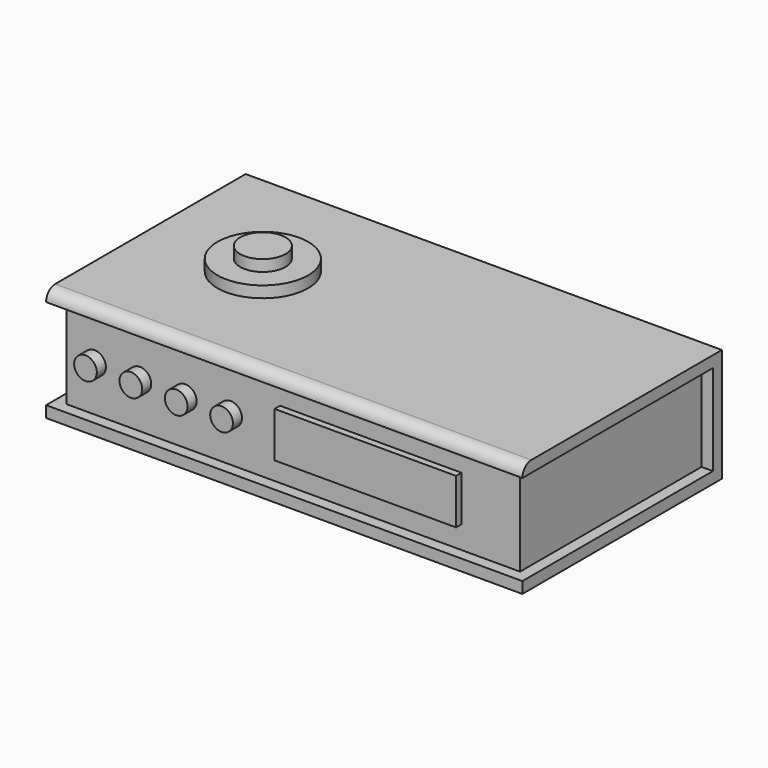
from build123d import *

# Parameters (mm, degrees)
F0_W      = 200
F0_H      = 100
F1_DEPTH  = 40
F2_W      = 210
F2_H      = 105
F2_W_2    = 200
F2_H_2    = 100
F3_DEPTH  = 5
F4_W      = 210
F4_H      = 105
F5_DEPTH  = 5
F6_W      = 210
F6_H      = 50
F7_DEPTH  = 5
F8_R      = 20
F9_DEPTH  = 5
F10_R     = 10
F11_DEPTH = 5
F12_R     = 5
F13_DEPTH = 5
F14_DEPTH = 5
F15_DEPTH = 5
F16_DEPTH = 5
F12_W     = 80
F12_H     = 20
F17_DEPTH = 3
F18_R     = 4.99999


# Not quite as in the source:
# - a fillet or chamfer is up to 0.001 mm smaller than in the source, because OpenCascade refuses the exact size


with BuildPart() as f1:
    # F0 (on Top) → F1 (new body)
    with BuildSketch(Plane.XY):
        with Locations((8.9475423098, -1.9630908966)):
            Rectangle(F0_W, F0_H)
    extrude(amount=F1_DEPTH)

    # F2 (on face) → F3 (join)
    with BuildSketch(Plane.XY.offset(40)):
        Polygon((113.9475423098, -56.9630908966), (113.9475423098, 48.0369091034), (108.9475423098, 48.0369091034), (108.9475423098, -51.9630908966), (-91.0524576902, -51.9630908966), (-91.0524576902, 48.0369091034), (-96.0524576902, 48.0369091034), (-96.0524576902, -56.9630908966), align=None)
        with Locations((8.9475423098, -4.4630908966)):
            Rectangle(F2_W, F2_H)
        with Locations((8.9475423098, -1.9630908966)):
            Rectangle(F2_W_2, F2_H_2)
    extrude(amount=F3_DEPTH)

    # F4 (on face) → F5 (join)
    with BuildSketch(Plane(origin=(0, 0, 0), x_dir=(1, 0, 0), z_dir=(0, 0, -1))):
        with Locations((8.9475423098, 4.4630908966)):
            Rectangle(F4_W, F4_H)
    extrude(amount=F5_DEPTH)

    # F6 (on face) → F7 (join)
    with BuildSketch(Plane(origin=(0, 48.0369091034, 0), x_dir=(-1, 0, 0), z_dir=(0, 1, 0))):
        with Locations((-8.9475423098, 20)):
            Rectangle(F6_W, F6_H)
    extrude(amount=F7_DEPTH)

    # F8 (on face) → F9 (join)
    with BuildSketch(Plane.XY.offset(45)):
        with Locations((-46.0524576902, 0)):
            Circle(F8_R)
    extrude(amount=F9_DEPTH)

    # F10 (on face) → F11 (join)
    with BuildSketch(Plane.XY.offset(50)):
        with Locations((-46.0524576902, 0)):
            Circle(F10_R)
    extrude(amount=F11_DEPTH)

    # F12 (on face) → F13 (join)
    with BuildSketch(Plane.XZ.offset(51.9630908966)):
        with Locations((-78.6770284176, 20)):
            Circle(F12_R)
    extrude(amount=F13_DEPTH)

    # F12 (on face) → F14 (join)
    with BuildSketch(Plane.XZ.offset(51.9630908966)):
        with Locations((-58.6770284176, 20)):
            Circle(F12_R)
    extrude(amount=F14_DEPTH)

    # F12 (on face) → F15 (join)
    with BuildSketch(Plane.XZ.offset(51.9630908966)):
        with Locations((-38.6770284176, 19.7612177581)):
            Circle(F12_R)
    extrude(amount=F15_DEPTH)

    # F12 (on face) → F16 (join)
    with BuildSketch(Plane.XZ.offset(51.9630908966)):
        with Locations((-18.6770284176, 19.7612177581)):
            Circle(F12_R)
    extrude(amount=F16_DEPTH)

    # F12 (on face) → F17 (join)
    with BuildSketch(Plane.XZ.offset(51.9630908966)):
        with Locations((43.1329405028, 20)):
            Rectangle(F12_W, F12_H)
    extrude(amount=F17_DEPTH)

    # F18 (radius 5 in the source; OpenCascade refuses exactly that, so slightly less here)
    f18_edges = [f1.edges().sort_by_distance(p)[0] for p in [
        (8.947542, -56.963091, 45),
    ]]
    fillet(f18_edges, radius=F18_R)


solid = f1.part
